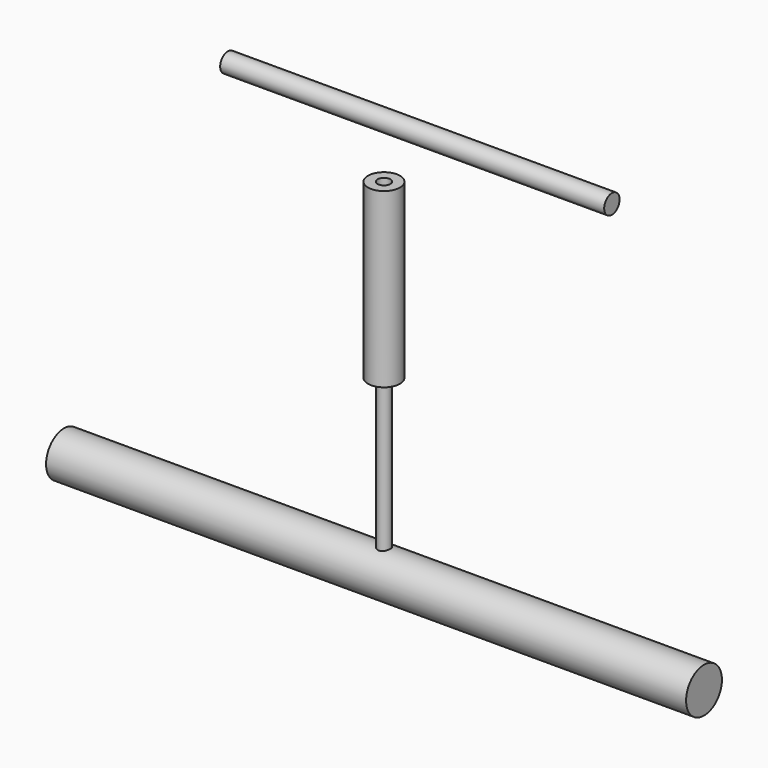
from build123d import *

# Parameters (mm, degrees)
F0_R     = 31.75
F0_R_2   = 12.7
F1_DEPTH = 342.9
F2_DEPTH = 304.8
F3_R     = 44.45
F4_DEPTH = 635
F5_DEPTH = 635
F6_R     = 19.05
F7_DEPTH = 381
F8_DEPTH = 381


with BuildPart() as f1:
    # F0 (on Top) → F1 (new body)
    with BuildSketch(Plane.XY):
        Circle(F0_R)
        Circle(F0_R_2, mode=Mode.SUBTRACT)
    extrude(amount=F1_DEPTH)


with BuildPart() as f2:
    # F0 (on Top) → F2 (new body)
    with BuildSketch(Plane.XY):
        Circle(F0_R_2)
    extrude(amount=-F2_DEPTH)


with BuildPart() as f4:
    # F3 (on Right) → F4 (new body)
    with BuildSketch(Plane.YZ):
        with Locations((0, -338.9594081884)):
            Circle(F3_R)
    extrude(amount=F4_DEPTH)

    # F3 (on Right) → F5 (join)
    with BuildSketch(Plane.YZ):
        with Locations((0, -338.9594081884)):
            Circle(F3_R)
    extrude(amount=-F5_DEPTH)


with BuildPart() as f7:
    # F6 (on Right) → F7 (new body)
    with BuildSketch(Plane.YZ):
        with Locations((88.997989893, 391.5736377239)):
            Circle(F6_R)
    extrude(amount=F7_DEPTH)

    # F6 (on Right) → F8 (join)
    with BuildSketch(Plane.YZ):
        with Locations((88.997989893, 391.5736377239)):
            Circle(F6_R)
    extrude(amount=-F8_DEPTH)


solid = Compound([f1.part, f2.part, f4.part, f7.part])
